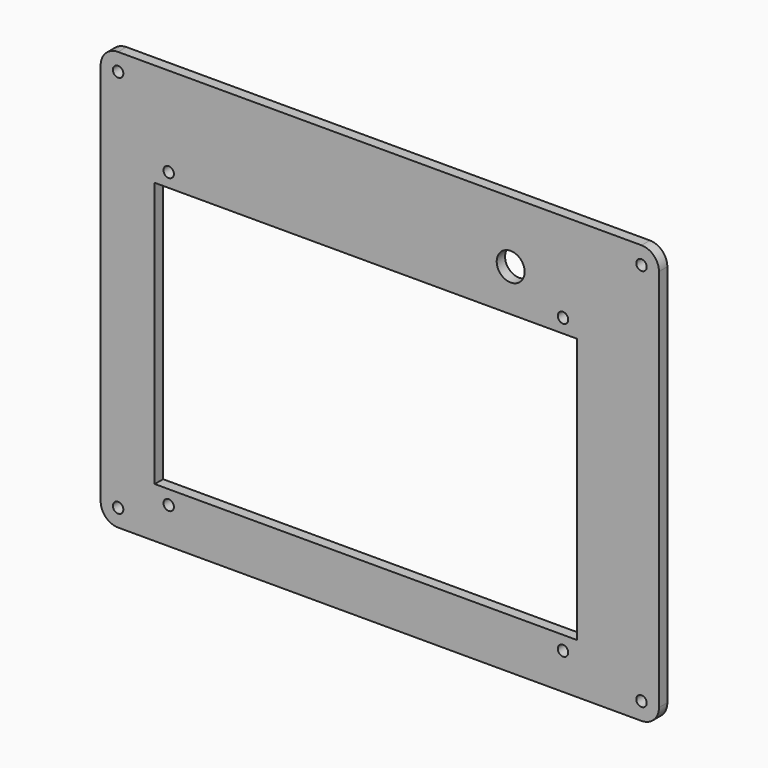
from build123d import *

# Parameters (mm, degrees)
F1_DEPTH = 3
F2_R     = 1.5
F3_DEPTH = 25
F4_R     = 1.5
F5_DEPTH = 25
F6_W     = 121
F6_H     = 76
F6_R     = 1.5
F7_DEPTH = 3
F8_R     = 4
F9_DEPTH = 3


# Not quite as in the source:
# - a feature names something its author has since deleted; it is built from what else it names


with BuildPart() as f1:
    # F0 (on Front) → F1 (new body)
    with BuildSketch(Plane.XZ):
        with BuildLine():
            Line((-75, -60), (75, -60))
            ThreePointArc((75, -60), (78.5355339059, -58.5355339059), (80, -55))
            Line((80, -55), (80, 55))
            ThreePointArc((80, 55), (78.5355339059, 58.5355339059), (75, 60))
            Line((75, 60), (-75, 60))
            ThreePointArc((-75, 60), (-78.5355339059, 58.5355339059), (-80, 55))
            Line((-80, 55), (-80, -55))
            ThreePointArc((-80, -55), (-78.5355339059, -58.5355339059), (-75, -60))
        make_face()
    extrude(amount=F1_DEPTH)

    # F2 (on Front) → F3 (cut)
    with BuildSketch(Plane.XZ):
        with Locations((-75, 55)):
            Circle(F2_R)
        with Locations((75, 55)):
            Circle(F2_R)
        with Locations((75, -55)):
            Circle(F2_R)
        with Locations((-75, -55)):
            Circle(F2_R)
    extrude(amount=F3_DEPTH, mode=Mode.SUBTRACT)

    # F4 (on Front) → F5 (cut)
    with BuildSketch(Plane.XZ):
        with Locations((52.5, 34.4)):
            Circle(F4_R)
    extrude(amount=F5_DEPTH, mode=Mode.SUBTRACT)

    # F6 (on face) → F7 (cut)
    with BuildSketch(Plane.XZ.offset(3)):
        with Locations((-4, -7.6)):
            Rectangle(F6_W, F6_H)
        with Locations((52.5, 34.4)):
            Circle(F6_R)
        with Locations((-60.5, 34.4)):
            Circle(F6_R)
        with Locations((-60.5, -49.6)):
            Circle(F6_R)
        with Locations((52.5, -49.6)):
            Circle(F6_R)
    extrude(amount=-F7_DEPTH, mode=Mode.SUBTRACT)

    # F8 (on face) → F9 (cut)
    with BuildSketch(Plane.XZ.offset(3)):
        with Locations((37.5, 42.4)):
            Circle(F8_R)
    extrude(amount=-F9_DEPTH, mode=Mode.SUBTRACT)


solid = f1.part
